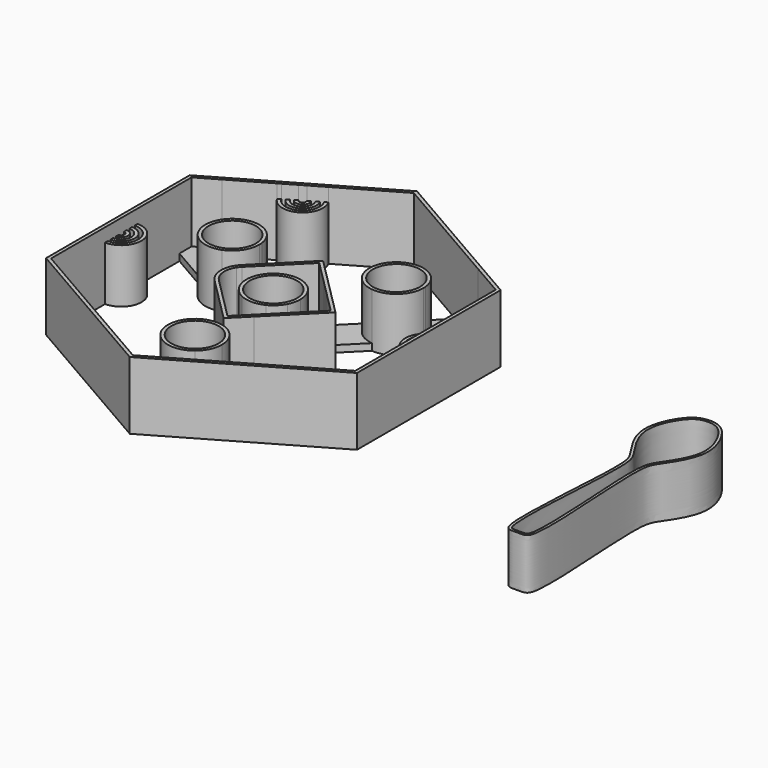
from build123d import *

# Parameters (mm, degrees)
F1_DEPTH = 15
F2_DEPTH = 20
F3_DEPTH = 16
F0_R     = 7
F4_DEPTH = 2


# Not quite as in the source:
# - the dataset's text gives a spline's control points without its knots; the knots are read off the source's solid


with BuildPart() as f1:
    # F0 (on Top) → F1 (new body)
    with BuildSketch(Plane.XY):
        with BuildLine():
            add(Edge.make_bspline(
                [(0, 35.8), (0.7513307109, 35.8), (2.1305033751, 35.6210703287), (3.8679092138, 34.805141972), (5.0496464599, 33.7475924076), (5.8950890437, 32.7290026602), (6.503377285, 31.8806920158), (7.0883693673, 30.9444653781), (7.8158917507, 29.5953080034), (8.5960708267, 27.7415773371), (9.1109074131, 25.7285174145), (9.3030526279, 24.0605541863), (9.3221306177, 22.7922621364), (9.1956178125, 21.5136552302), (8.9252996726, 20.2634346664), (8.5421398673, 19.0485253443), (7.9119194269, 17.4840824015), (6.9603187706, 15.647901981), (5.9410115143, 14.0160529673), (5.1750330978, 12.8657953253), (4.6475686608, 12.0889369837), (4.1938233257, 11.4139450752), (3.6923873768, 10.614706158), (3.3316815221, 9.8926569974), (3.0623334456, 9.0521120168), (2.8995595302, 8.3076755124), (2.7750179718, 7.4002488529), (2.6882537775, 6.3031220091), (2.6380950188, 5.0441202156), (2.6161143168, 3.1711435065), (2.6644765482, 0.5083066043), (2.8145360242, -3.0781816874), (3.0263714652, -6.9369532248), (3.2694986904, -10.9511857046), (3.5136352386, -15.0049232352), (3.7274467694, -18.9838415737), (3.8836209117, -22.7708242689), (3.967026188, -26.2524114354), (3.9616553045, -28.8064833496), (3.9036016999, -30.5885013887), (3.8306191818, -31.7825340023), (3.7249586242, -32.824074757), (3.6056057177, -33.5599688317), (3.4852718702, -34.0721515509), (3.3783205862, -34.4215823165), (3.2490822984, -34.7404594703), (3.068094238, -35.0548744216), (2.8026439636, -35.3469947914), (2.4653346363, -35.5639409031), (2.1118742358, -35.6891481042), (1.7609239162, -35.7539719967), (1.3958233928, -35.7853932502), (0.8612749968, -35.8022854934), (0.3778354732, -35.8), (0, -35.8)],
                knots=[0, 0, 0, 0, 0.03125, 0.0625, 0.09375, 0.109375, 0.125, 0.140625, 0.15625, 0.1875, 0.21875, 0.234375, 0.25, 0.265625, 0.28125, 0.296875, 0.3125, 0.34375, 0.375, 0.390625, 0.40625, 0.421875, 0.4375, 0.46875, 0.484375, 0.5, 0.515625, 0.53125, 0.546875, 0.5625, 0.59375, 0.625, 0.65625, 0.6875, 0.71875, 0.75, 0.78125, 0.8125, 0.84375, 0.859375, 0.875, 0.890625, 0.90625, 0.9140625, 0.921875, 0.9296875, 0.9375, 0.9453125, 0.953125, 0.9609375, 0.96875, 0.9765625, 0.984375, 1, 1, 1, 1], degree=3))
            add(Edge.make_bspline(
                [(0, 35.8), (-0.7513307109, 35.8), (-2.1305033751, 35.6210703287), (-3.8679092138, 34.805141972), (-5.0496464599, 33.7475924076), (-5.8950890437, 32.7290026602), (-6.503377285, 31.8806920158), (-7.0883693673, 30.9444653781), (-7.8158917507, 29.5953080034), (-8.5960708267, 27.7415773371), (-9.1109074131, 25.7285174145), (-9.3030526279, 24.0605541863), (-9.3221306177, 22.7922621364), (-9.1956178125, 21.5136552302), (-8.9252996726, 20.2634346664), (-8.5421398673, 19.0485253443), (-7.9119194269, 17.4840824015), (-6.9603187706, 15.647901981), (-5.9410115143, 14.0160529673), (-5.1750330978, 12.8657953253), (-4.6475686608, 12.0889369837), (-4.1938233257, 11.4139450752), (-3.6923873768, 10.614706158), (-3.3316815221, 9.8926569974), (-3.0623334456, 9.0521120168), (-2.8995595302, 8.3076755124), (-2.7750179718, 7.4002488529), (-2.6882537775, 6.3031220091), (-2.6380950188, 5.0441202156), (-2.6161143168, 3.1711435065), (-2.6644765482, 0.5083066043), (-2.8145360242, -3.0781816874), (-3.0263714652, -6.9369532248), (-3.2694986904, -10.9511857046), (-3.5136352386, -15.0049232352), (-3.7274467694, -18.9838415737), (-3.8836209117, -22.7708242689), (-3.967026188, -26.2524114354), (-3.9616553045, -28.8064833496), (-3.9036016999, -30.5885013887), (-3.8306191818, -31.7825340023), (-3.7249586242, -32.824074757), (-3.6056057177, -33.5599688317), (-3.4852718702, -34.0721515509), (-3.3783205862, -34.4215823165), (-3.2490822984, -34.7404594703), (-3.068094238, -35.0548744216), (-2.8026439636, -35.3469947914), (-2.4653346363, -35.5639409031), (-2.1118742358, -35.6891481042), (-1.7609239162, -35.7539719967), (-1.3958233928, -35.7853932502), (-0.8612749968, -35.8022854934), (-0.3778354732, -35.8), (0, -35.8)],
                knots=[0, 0, 0, 0, 0.03125, 0.0625, 0.09375, 0.109375, 0.125, 0.140625, 0.15625, 0.1875, 0.21875, 0.234375, 0.25, 0.265625, 0.28125, 0.296875, 0.3125, 0.34375, 0.375, 0.390625, 0.40625, 0.421875, 0.4375, 0.46875, 0.484375, 0.5, 0.515625, 0.53125, 0.546875, 0.5625, 0.59375, 0.625, 0.65625, 0.6875, 0.71875, 0.75, 0.78125, 0.8125, 0.84375, 0.859375, 0.875, 0.890625, 0.90625, 0.9140625, 0.921875, 0.9296875, 0.9375, 0.9453125, 0.953125, 0.9609375, 0.96875, 0.9765625, 0.984375, 1, 1, 1, 1], degree=3))
        make_face()
        with BuildLine():
            add(Edge.make_bspline(
                [(0, 35), (-2.4821149589, 35), (-5.9402523615, 32.5500189943), (-10.5337777253, 21.9192868933), (-3.7192044125, 12.2544173944), (-0.9843000607, 7.8359148369), (-3.1441119834, -17.1474175153), (-3.3835196014, -35.1096976257), (-1.8110210273, -35), (0, -35)],
                knots=[0, 0, 0, 0, 0.1127387007, 0.2598296767, 0.4081784934, 0.5105364273, 0.7413956382, 0.9254919835, 1, 1, 1, 1], degree=3))
            add(Edge.make_bspline(
                [(0, 35), (2.4821149589, 35), (5.9402523615, 32.5500189943), (10.5337777253, 21.9192868933), (3.7192044125, 12.2544173944), (0.9843000607, 7.8359148369), (3.1441119834, -17.1474175153), (3.3835196014, -35.1096976257), (1.8110210273, -35), (0, -35)],
                knots=[0, 0, 0, 0, 0.1127387007, 0.2598296767, 0.4081784934, 0.5105364273, 0.7413956382, 0.9254919835, 1, 1, 1, 1], degree=3))
        make_face(mode=Mode.SUBTRACT)
    extrude(amount=-F1_DEPTH)


with BuildPart() as f2:
    # F0 (on Top) → F2 (new body)
    with BuildSketch(Plane.XY):
        Polygon((-146.6593033671, 26.5581123827), (-146.6593033671, -26.5581123827), (-100.6593033671, -53.1162247654), (-54.6593033671, -26.5581123827), (-54.6593033671, 26.5581123827), (-100.6593033671, 53.1162247654), align=None)
        Polygon((-145.6593033671, 21.5078068853), (-145.6593033671, 25.9807621135), (-139.5329947833, 29.5177880235), (-128.3554557898, 35.9711431703), (-127.4894303861, 36.4711431703), (-126.6234049823, 36.9711431703), (-125.7573795785, 37.4711431703), (-124.8913541747, 37.9711431703), (-124.0253287709, 38.4711431703), (-122.2932779634, 39.4711431703), (-121.4272525596, 39.9711431703), (-120.5612271558, 40.4711431703), (-119.695201752, 40.9711431703), (-118.8291763482, 41.4711431703), (-117.9631509444, 41.9711431703), (-100.6593033671, 51.9615242271), (-74.4573358451, 36.8338112249), (-65.4915830423, 31.6574314307), (-55.6593033671, 25.9807621135), (-55.6593033671, 6), (-55.6593033671, 5), (-55.6593033671, 4), (-55.6593033671, 3), (-55.6593033671, 2), (-55.6593033671, 1), (-55.6593033671, -1), (-55.6593033671, -2), (-55.6593033671, -3), (-55.6593033671, -4), (-55.6593033671, -5), (-55.6593033671, -6), (-55.6593033671, -25.9807621135), (-72.9631509444, -35.9711431703), (-73.8291763482, -36.4711431703), (-74.695201752, -36.9711431703), (-75.5612271558, -37.4711431703), (-76.4272525596, -37.9711431703), (-77.2932779634, -38.4711431703), (-79.0253287709, -39.4711431703), (-79.8913541747, -39.9711431703), (-80.7573795785, -40.4711431703), (-81.6234049823, -40.9711431703), (-82.4894303861, -41.4711431703), (-83.3554557898, -41.9711431703), (-95.6593006849, -49.0747713325), (-100.6593033671, -51.9615242271), (-105.6593033671, -49.0747728811), (-145.6593033671, -25.9807621135), (-145.6593033671, -6), (-145.6593033671, -5), (-145.6593033671, -4), (-145.6593033671, -3), (-145.6593033671, -2), (-145.6593033671, -1), (-145.6593033671, 1), (-145.6593033671, 2), (-145.6593033671, 3), (-145.6593033671, 4), (-145.6593033671, 5), (-145.6593033671, 6), align=None, mode=Mode.SUBTRACT)
    extrude(amount=F2_DEPTH)

    # F0 (on Top) → F3 (join)
    with BuildSketch(Plane.XY):
        with BuildLine():
            Line((-127.4894303861, 36.4711431703), (-128.3554557898, 35.9711431703))
            ThreePointArc((-128.3554557898, 35.9711431703), (-120.1593033671, 33.7749907476), (-117.9631509444, 41.9711431703))
            Line((-117.9631509444, 41.9711431703), (-118.8291763482, 41.4711431703))
            ThreePointArc((-118.8291763482, 41.4711431703), (-120.6593033671, 34.6410161514), (-127.4894303861, 36.4711431703))
        make_face()
        with BuildLine():
            Line((-125.7573795785, 37.4711431703), (-126.6234049823, 36.9711431703))
            ThreePointArc((-126.6234049823, 36.9711431703), (-121.1593033671, 35.5070415552), (-119.695201752, 40.9711431703))
            Line((-119.695201752, 40.9711431703), (-120.5612271558, 40.4711431703))
            ThreePointArc((-120.5612271558, 40.4711431703), (-121.6593033671, 36.3730669589), (-125.7573795785, 37.4711431703))
        make_face()
        with BuildLine():
            Line((-124.0253287709, 38.4711431703), (-124.8913541747, 37.9711431703))
            ThreePointArc((-124.8913541747, 37.9711431703), (-122.1593033671, 37.2390923627), (-121.4272525596, 39.9711431703))
            Line((-121.4272525596, 39.9711431703), (-122.2932779634, 39.4711431703))
            ThreePointArc((-122.2932779634, 39.4711431703), (-122.6593033671, 38.1051177665), (-124.0253287709, 38.4711431703))
        make_face()
        with BuildLine():
            ThreePointArc((-145.6593033671, -6), (-139.6593033671, 0), (-145.6593033671, 6))
            Line((-145.6593033671, 6), (-145.6593033671, 5))
            ThreePointArc((-145.6593033671, 5), (-140.6593033671, 0), (-145.6593033671, -5))
            Line((-145.6593033671, -5), (-145.6593033671, -6))
        make_face()
        with BuildLine():
            ThreePointArc((-145.6593033671, -4), (-141.6593033671, 0), (-145.6593033671, 4))
            Line((-145.6593033671, 4), (-145.6593033671, 3))
            ThreePointArc((-145.6593033671, 3), (-142.6593033671, 0), (-145.6593033671, -3))
            Line((-145.6593033671, -3), (-145.6593033671, -4))
        make_face()
        with BuildLine():
            ThreePointArc((-145.6593033671, -2), (-143.6593033671, 0), (-145.6593033671, 2))
            Line((-145.6593033671, 2), (-145.6593033671, 1))
            ThreePointArc((-145.6593033671, 1), (-144.6593033671, 0), (-145.6593033671, -1))
            Line((-145.6593033671, -1), (-145.6593033671, -2))
        make_face()
        with BuildLine():
            ThreePointArc((-72.9631509444, -35.9711431703), (-81.1593033671, -33.7749907476), (-83.3554557898, -41.9711431703))
            Line((-83.3554557898, -41.9711431703), (-82.4894303861, -41.4711431703))
            ThreePointArc((-82.4894303861, -41.4711431703), (-80.6593033671, -34.6410161514), (-73.8291763482, -36.4711431703))
            Line((-73.8291763482, -36.4711431703), (-72.9631509444, -35.9711431703))
        make_face()
        with BuildLine():
            ThreePointArc((-74.695201752, -36.9711431703), (-80.1593033671, -35.5070415552), (-81.6234049823, -40.9711431703))
            Line((-81.6234049823, -40.9711431703), (-80.7573795785, -40.4711431703))
            ThreePointArc((-80.7573795785, -40.4711431703), (-79.6593033671, -36.3730669589), (-75.5612271558, -37.4711431703))
            Line((-75.5612271558, -37.4711431703), (-74.695201752, -36.9711431703))
        make_face()
        with BuildLine():
            ThreePointArc((-76.4272525596, -37.9711431703), (-79.1593033671, -37.2390923627), (-79.8913541747, -39.9711431703))
            Line((-79.8913541747, -39.9711431703), (-79.0253287709, -39.4711431703))
            ThreePointArc((-79.0253287709, -39.4711431703), (-78.6593033671, -38.1051177665), (-77.2932779634, -38.4711431703))
            Line((-77.2932779634, -38.4711431703), (-76.4272525596, -37.9711431703))
        make_face()
        with BuildLine():
            Line((-55.6593033671, 5), (-55.6593033671, 6))
            ThreePointArc((-55.6593033671, 6), (-61.6593033671, 0), (-55.6593033671, -6))
            Line((-55.6593033671, -6), (-55.6593033671, -5))
            ThreePointArc((-55.6593033671, -5), (-60.6593033671, 0), (-55.6593033671, 5))
        make_face()
        with BuildLine():
            Line((-55.6593033671, 3), (-55.6593033671, 4))
            ThreePointArc((-55.6593033671, 4), (-59.6593033671, 0), (-55.6593033671, -4))
            Line((-55.6593033671, -4), (-55.6593033671, -3))
            ThreePointArc((-55.6593033671, -3), (-58.6593033671, 0), (-55.6593033671, 3))
        make_face()
        with BuildLine():
            Line((-55.6593033671, 1), (-55.6593033671, 2))
            ThreePointArc((-55.6593033671, 2), (-57.6593033671, 0), (-55.6593033671, -2))
            Line((-55.6593033671, -2), (-55.6593033671, -1))
            ThreePointArc((-55.6593033671, -1), (-56.6593033671, 0), (-55.6593033671, 1))
        make_face()
    extrude(amount=F3_DEPTH)



with BuildPart() as f3:
    # F0 (on Top) → F3, piece 2 (new body)
    with BuildSketch(Plane.XY):
        with BuildLine():
            ThreePointArc((-117.2836111381, 16.6721003866), (-121.1919377725, 22.3926737719), (-128.1002629656, 22.917097231))
            ThreePointArc((-128.1002629656, 22.917097231), (-132.1201405412, 19.4644713411), (-133.1002646857, 14.2568425219))
            ThreePointArc((-133.1002646857, 14.2568425219), (-129.1919377725, 8.5362673113), (-122.2836108593, 8.0118445235))
            ThreePointArc((-122.2836108593, 8.0118445235), (-118.5863864971, 10.9515233508), (-117.1919377725, 15.4644705416))
            ThreePointArc((-117.1919377725, 15.4644705416), (-117.2148890364, 16.0700227376), (-117.2836111381, 16.6721003866))
        make_face()
        with Locations((-125.1919377725, 15.4644705416)):
            Circle(F0_R, mode=Mode.SUBTRACT)
    extrude(amount=F3_DEPTH)


with BuildPart() as f3b:
    # F0 (on Top) → F3, piece 3 (new body)
    with BuildSketch(Plane.XY):
        with BuildLine():
            ThreePointArc((-74.0596155774, 23.0893988956), (-76.3541763346, 27.8659048621), (-81.1306830876, 30.1604639824))
            ThreePointArc((-81.1306830876, 30.1604639824), (-87.6678838643, 27.8659038928), (-89.9624439539, 21.3287031161))
            ThreePointArc((-89.9624439539, 21.3287031161), (-87.6678848336, 16.5521963631), (-82.8913788671, 14.2576356059))
            ThreePointArc((-82.8913788671, 14.2576356059), (-76.6744948786, 16.2490666727), (-74.0110296148, 22.2090496433))
            ThreePointArc((-74.0110296148, 22.2090496433), (-74.0231853406, 22.6498941175), (-74.0596155774, 23.0893988956))
        make_face()
        with Locations((-82.0110296148, 22.2090496433)):
            Circle(F0_R, mode=Mode.SUBTRACT)
    extrude(amount=F3_DEPTH)


with BuildPart() as f3c:
    # F0 (on Top) → F3, piece 4 (new body)
    with BuildSketch(Plane.XY):
        with BuildLine():
            Line((-100.6593033671, 18.3847763109), (-107.8300153591, 11.2140643189))
            Line((-107.8300153591, 11.2140643189), (-114.0943322097, 4.9497474683))
            ThreePointArc((-114.0943322097, 4.9497474683), (-114.5837883481, 4.4062528439), (-115.013862401, 3.8146532941))
            ThreePointArc((-115.013862401, 3.8146532941), (-116.1063737615, -0.7304064891), (-114.0943322097, -4.9497474683))
            Line((-114.0943322097, -4.9497474683), (-105.6593033671, -13.3847763109))
            Line((-105.6593033671, -13.3847763109), (-100.6593033671, -18.3847763109))
            Line((-100.6593033671, -18.3847763109), (-95.6593006849, -13.3847736286))
            Line((-95.6593006849, -13.3847736286), (-82.2745270563, 0))
            Line((-82.2745270563, 0), (-89.7117707646, 7.4372437083))
            Line((-89.7117707646, 7.4372437083), (-96.7828370631, 14.5083100068))
            Line((-96.7828370631, 14.5083100068), (-100.6593033671, 18.3847763109))
        make_face()
        with BuildLine():
            ThreePointArc((-113.3872254285, -4.2426406871), (-115.114529034, -0.5998042544), (-114.14643015, 3.3138410505))
            ThreePointArc((-114.14643015, 3.3138410505), (-113.7900984896, 3.7972624369), (-113.3872254285, 4.2426406871))
            Line((-113.3872254285, 4.2426406871), (-110.9123516943, 6.7175144213))
            Line((-110.9123516943, 6.7175144213), (-107.3768177884, 10.2530483272))
            Line((-107.3768177884, 10.2530483272), (-100.6593033671, 16.9705627485))
            Line((-100.6593033671, 16.9705627485), (-93.9417889459, 10.2530483272))
            Line((-93.9417889459, 10.2530483272), (-90.4062550399, 6.7175144213))
            Line((-90.4062550399, 6.7175144213), (-83.6887406187, 0))
            Line((-83.6887406187, 0), (-90.4062550399, -6.7175144213))
            Line((-90.4062550399, -6.7175144213), (-93.9417889459, -10.2530483272))
            Line((-93.9417889459, -10.2530483272), (-100.6593033671, -16.9705627485))
            Line((-100.6593033671, -16.9705627485), (-107.3768177884, -10.2530483272))
            Line((-107.3768177884, -10.2530483272), (-110.9123516943, -6.7175144213))
            Line((-110.9123516943, -6.7175144213), (-113.3872254285, -4.2426406871))
        make_face(mode=Mode.SUBTRACT)
    extrude(amount=F3_DEPTH)


with BuildPart() as f3d:
    # F0 (on Top) → F3, piece 5 (new body)
    with BuildSketch(Plane.XY):
        with BuildLine():
            ThreePointArc((-105.6593033671, -22.7550020016), (-108.6593033671, -29), (-105.6593033671, -35.2449979984))
            ThreePointArc((-105.6593033671, -35.2449979984), (-100.6593016491, -37), (-95.6593006849, -35.2449958509))
            ThreePointArc((-95.6593006849, -35.2449958509), (-93.4482000723, -32.4641000666), (-92.6593033671, -29))
            ThreePointArc((-92.6593033671, -29), (-93.4482000723, -25.5358999334), (-95.6593006849, -22.7550041491))
            ThreePointArc((-95.6593006849, -22.7550041491), (-100.6593016491, -21), (-105.6593033671, -22.7550020016))
        make_face()
        with Locations((-100.6593033671, -29)):
            Circle(F0_R, mode=Mode.SUBTRACT)
    extrude(amount=F3_DEPTH)


with BuildPart() as f3e:
    # F0 (on Top) → F3, piece 6 (new body)
    with BuildSketch(Plane.XY):
        with BuildLine():
            ThreePointArc((-104.2650827292, 7.141313268), (-106.3161576166, 5.6568542495), (-107.8006166352, 3.6057793621))
            ThreePointArc((-107.8006166352, 3.6057793621), (-108.6593033671, 0), (-107.8006166352, -3.6057793621))
            ThreePointArc((-107.8006166352, -3.6057793621), (-106.3161576166, -5.6568542495), (-104.2650827292, -7.141313268))
            ThreePointArc((-104.2650827292, -7.141313268), (-100.6593033671, -8), (-97.0535240051, -7.141313268))
            ThreePointArc((-97.0535240051, -7.141313268), (-95.0024491176, -5.6568542495), (-93.5179900991, -3.6057793621))
            ThreePointArc((-93.5179900991, -3.6057793621), (-92.8769352782, -1.8533070247), (-92.6593033671, 0))
            ThreePointArc((-92.6593033671, 0), (-92.8769352782, 1.8533070247), (-93.5179900991, 3.6057793621))
            ThreePointArc((-93.5179900991, 3.6057793621), (-95.0024491176, 5.6568542495), (-97.0535240051, 7.141313268))
            ThreePointArc((-97.0535240051, 7.141313268), (-100.6593033671, 8), (-104.2650827292, 7.141313268))
        make_face()
        with Locations((-100.6593033671, 0)):
            Circle(F0_R, mode=Mode.SUBTRACT)
    extrude(amount=F3_DEPTH)


with BuildPart() as f2_1:
    add(f2.part)

    add(f3.part)  # F4 merges F3

    add(f3b.part)  # F4 merges F3b

    add(f3c.part)  # F4 merges F3c

    add(f3d.part)  # F4 merges F3d

    add(f3e.part)  # F4 merges F3e
    # F0 (on Top) → F4 (join)
    with BuildSketch(Plane.XY):
        with BuildLine():
            Line((-139.5329947833, 29.5177880235), (-145.6593033671, 25.9807621135))
            Line((-145.6593033671, 25.9807621135), (-145.6593033671, 21.5078068853))
            Line((-145.6593033671, 21.5078068853), (-133.1002646857, 14.2568425219))
            ThreePointArc((-133.1002646857, 14.2568425219), (-132.1201405412, 19.4644713411), (-128.1002629656, 22.917097231))
            Line((-128.1002629656, 22.917097231), (-139.5329947833, 29.5177880235))
        make_face()
        with BuildLine():
            Line((-107.8300153591, 11.2140643189), (-117.2836111381, 16.6721003866))
            ThreePointArc((-117.2836111381, 16.6721003866), (-117.2148890364, 16.0700227376), (-117.1919377725, 15.4644705416))
            ThreePointArc((-117.1919377725, 15.4644705416), (-118.5863864971, 10.9515233508), (-122.2836108593, 8.0118445235))
            Line((-122.2836108593, 8.0118445235), (-115.013862401, 3.8146532941))
            ThreePointArc((-115.013862401, 3.8146532941), (-114.5837883481, 4.4062528439), (-114.0943322097, 4.9497474683))
            Line((-114.0943322097, 4.9497474683), (-107.8300153591, 11.2140643189))
        make_face()
        with BuildLine():
            Line((-89.9624439539, 21.3287031161), (-96.7828370631, 14.5083100068))
            Line((-96.7828370631, 14.5083100068), (-89.7117707646, 7.4372437083))
            Line((-89.7117707646, 7.4372437083), (-82.8913788671, 14.2576356059))
            ThreePointArc((-82.8913788671, 14.2576356059), (-87.6678848336, 16.5521963631), (-89.9624439539, 21.3287031161))
        make_face()
        with BuildLine():
            Line((-65.4915830423, 31.6574314307), (-74.4573358451, 36.8338112249))
            Line((-74.4573358451, 36.8338112249), (-81.1306830876, 30.1604639824))
            ThreePointArc((-81.1306830876, 30.1604639824), (-76.3541763346, 27.8659048621), (-74.0596155774, 23.0893988956))
            Line((-74.0596155774, 23.0893988956), (-65.4915830423, 31.6574314307))
        make_face()
        with BuildLine():
            Line((-100.6593033671, -18.3847763109), (-105.6593033671, -13.3847763109))
            Line((-105.6593033671, -13.3847763109), (-105.6593033671, -22.7550020016))
            ThreePointArc((-105.6593033671, -22.7550020016), (-100.6593016491, -21), (-95.6593006849, -22.7550041491))
            Line((-95.6593006849, -22.7550041491), (-95.6593006849, -13.3847736286))
            Line((-95.6593006849, -13.3847736286), (-100.6593033671, -18.3847763109))
        make_face()
        with BuildLine():
            Line((-105.6593033671, -35.2449979984), (-105.6593033671, -49.0747728811))
            Line((-105.6593033671, -49.0747728811), (-100.6593033671, -51.9615242271))
            Line((-100.6593033671, -51.9615242271), (-95.6593006849, -49.0747713325))
            Line((-95.6593006849, -49.0747713325), (-95.6593006849, -35.2449958509))
            ThreePointArc((-95.6593006849, -35.2449958509), (-100.6593016491, -37), (-105.6593033671, -35.2449979984))
        make_face()
        with BuildLine():
            Line((-107.8006166352, -3.6057793621), (-110.9123516943, -6.7175144213))
            Line((-110.9123516943, -6.7175144213), (-107.3768177884, -10.2530483272))
            Line((-107.3768177884, -10.2530483272), (-104.2650827292, -7.141313268))
            ThreePointArc((-104.2650827292, -7.141313268), (-106.3161576166, -5.6568542495), (-107.8006166352, -3.6057793621))
        make_face()
        with BuildLine():
            Line((-107.3768177884, 10.2530483272), (-110.9123516943, 6.7175144213))
            Line((-110.9123516943, 6.7175144213), (-107.8006166352, 3.6057793621))
            ThreePointArc((-107.8006166352, 3.6057793621), (-106.3161576166, 5.6568542495), (-104.2650827292, 7.141313268))
            Line((-104.2650827292, 7.141313268), (-107.3768177884, 10.2530483272))
        make_face()
        with BuildLine():
            Line((-90.4062550399, 6.7175144213), (-93.9417889459, 10.2530483272))
            Line((-93.9417889459, 10.2530483272), (-97.0535240051, 7.141313268))
            ThreePointArc((-97.0535240051, 7.141313268), (-95.0024491176, 5.6568542495), (-93.5179900991, 3.6057793621))
            Line((-93.5179900991, 3.6057793621), (-90.4062550399, 6.7175144213))
        make_face()
        with BuildLine():
            Line((-97.0535240051, -7.141313268), (-93.9417889459, -10.2530483272))
            Line((-93.9417889459, -10.2530483272), (-90.4062550399, -6.7175144213))
            Line((-90.4062550399, -6.7175144213), (-93.5179900991, -3.6057793621))
            ThreePointArc((-93.5179900991, -3.6057793621), (-95.0024491176, -5.6568542495), (-97.0535240051, -7.141313268))
        make_face()
    extrude(amount=F4_DEPTH)


solid = Compound([f1.part, f2_1.part])
